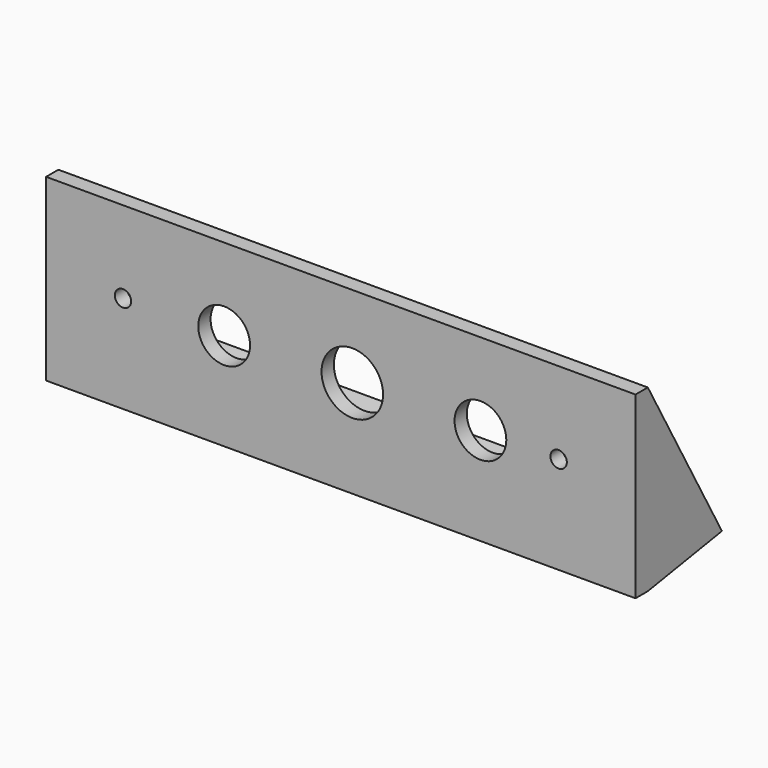
from build123d import *

# Parameters (mm, degrees)
F0_W     = 115
F0_H     = 35
F0_R     = 1.6
F0_R_2   = 5.05
F0_R_3   = 6
F1_DEPTH = 3
F3_DEPTH = 3
F5_DEPTH = 3
F7_DEPTH = 112
F8_R     = 2.1
F9_DEPTH = 4.2023227536


with BuildPart() as f1:
    # F0 (on Front) → F1 (new body)
    with BuildSketch(Plane.XZ):
        with Locations((-2.2430759668, 17.5)):
            Rectangle(F0_W, F0_H)
        with Locations((-44.7430759668, 19)):
            Circle(F0_R, mode=Mode.SUBTRACT)
        with Locations((-25, 19)):
            Circle(F0_R_2, mode=Mode.SUBTRACT)
        with Locations((0, 19)):
            Circle(F0_R_3, mode=Mode.SUBTRACT)
        with Locations((25, 19)):
            Circle(F0_R_2, mode=Mode.SUBTRACT)
        with Locations((40.2569240332, 19)):
            Circle(F0_R, mode=Mode.SUBTRACT)
    extrude(amount=F1_DEPTH)

    # F2 (on face) → F3 (join)
    with BuildSketch(Plane(origin=(-59.7430759668, 0, 0), x_dir=(0, -1, 0), z_dir=(-1, 0, 0))):
        Polygon((0, 0), (0, 35), (-17.954993993, 2.8193253092), align=None)
    extrude(amount=-F3_DEPTH)

    # F4 (on face) → F5 (join)
    with BuildSketch(Plane.YZ.offset(55.2569240332)):
        Polygon((18.0769208819, 2.9807693791), (0, 35), (0, 0), align=None)
    extrude(amount=-F5_DEPTH)

    # F6 (on face) → F7 (join)
    with BuildSketch(Plane(origin=(52.2569240332, 0, 0), x_dir=(0, -1, 0), z_dir=(-1, 0, 0))):
        Polygon((-17.4172232201, 4.1492765441), (-18.0769208819, 2.9807693791), (0, 0), (0, 1.2772871172), align=None)
    extrude(amount=F7_DEPTH)

    # F8 (on face) → F9 (cut, through all)
    with BuildSketch(Plane(origin=(0, -0.2050414688, 1.243477082), x_dir=(1, 0, 0), z_dir=(0, -0.1626966256, 0.9866761414))):
        with Locations((40.5074283481, 11.60009671)):
            Circle(F8_R)
        with Locations((-44.4925716519, 11.60009671)):
            Circle(F8_R)
    extrude(amount=-F9_DEPTH, mode=Mode.SUBTRACT)


solid = f1.part
